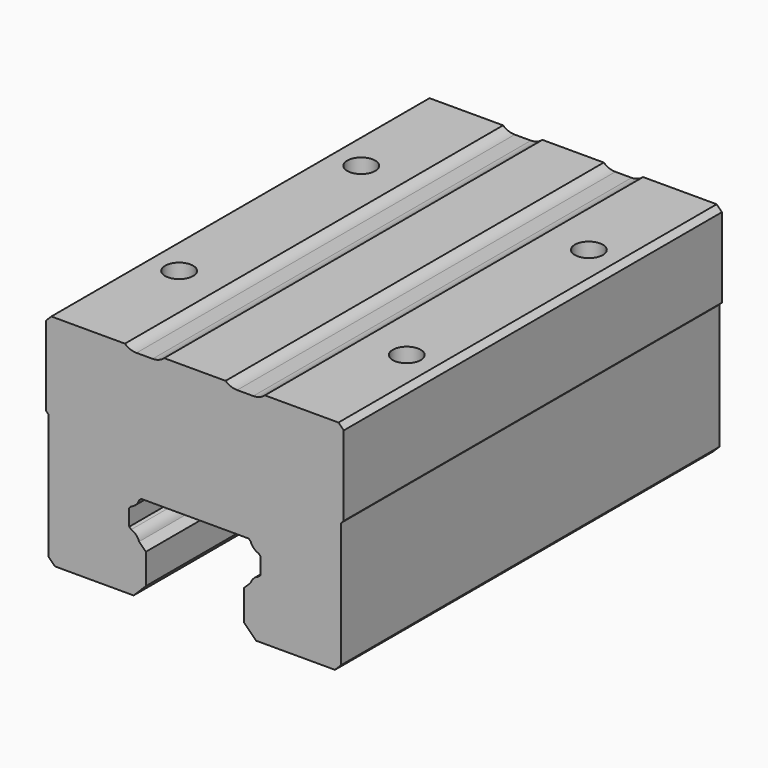
from build123d import *

# Parameters (mm, degrees)
F1_DEPTH = 54
F2_DEPTH = 54
F4_D     = 3.2
F4_DEPTH = 14.25
F4_TIP   = 0.9613769904


# Not quite as in the source:
# - ends of sketch curves that miss each other by under 0.0002 mm in the source are joined


with BuildPart() as f1:
    # F0 (on Front) → F1 (new body)
    with BuildSketch(Plane.XZ):
        with BuildLine():
            Line((-15.9999975914, -11.0858444687), (-13.9999981419, -11.0858444687))
            Line((-13.9999981419, -11.0858444687), (-14.9999975913, -10.0858455697))
            Line((-14.9999975913, -10.0858455697), (-14.9999975913, 8.4141544303))
            Line((-14.9999975913, 8.4141544303), (-13.9999975913, 9.4141544303))
            Line((-13.9999975913, 9.4141544303), (14.0000024087, 9.4141544303))
            Line((14.0000024087, 9.4141544303), (15.0000024087, 8.4141544303))
            Line((15.0000024087, 8.4141544303), (15.0000024087, -10.0858455697))
            Line((15.0000024087, -10.0858455697), (14.0000024087, -11.0858455697))
            Line((14.0000024087, -11.0858455697), (16.0000024087, -11.0858444685))
            Line((16.0000024087, -11.0858444685), (16.7000024086, -10.3858444685))
            Line((16.7000024086, -10.3858444685), (16.7000024087, 3.914155003))
            Line((16.7000024087, 3.914155003), (17.0000024087, 4.2141550029))
            Line((17.0000024087, 4.2141550029), (17.0000024088, 13.3141544304))
            Line((17.0000024088, 13.3141544304), (16.4000024089, 13.9141544303))
            Line((16.4000024089, 13.9141544303), (7.9944513482, 13.9141544304))
            ThreePointArc((7.9944513482, 13.9141544304), (7.3786811713, 13.5433235007), (6.671572232, 13.4141513784))
            Line((6.671572232, 13.4141513784), (4.8284325856, 13.4141513784))
            ThreePointArc((4.8284325856, 13.4141513784), (4.1213236463, 13.5433235007), (3.5055534694, 13.9141544304))
            Line((3.5055534694, 13.9141544304), (-3.5055486519, 13.9141544303))
            ThreePointArc((-3.5055486519, 13.9141544303), (-4.1213188288, 13.5433235006), (-4.828427768, 13.4141513784))
            Line((-4.828427768, 13.4141513784), (-6.6715674144, 13.4141513784))
            ThreePointArc((-6.6715674144, 13.4141513784), (-7.3788732943, 13.5428024468), (-7.9944465306, 13.9141544304))
            Line((-7.9944465306, 13.9141544304), (-16.3999975914, 13.9141544303))
            Line((-16.3999975914, 13.9141544303), (-16.9999975913, 13.3141544304))
            Line((-16.9999975913, 13.3141544304), (-16.9999975913, 4.2141550029))
            Line((-16.9999975913, 4.2141550029), (-16.6999975912, 3.9141550028))
            Line((-16.6999975912, 3.9141550028), (-16.6999975914, -10.3858444687))
            Line((-16.6999975914, -10.3858444687), (-15.9999975914, -11.0858444687))
        make_face()
    extrude(amount=-F1_DEPTH)

    # F0 (on Front) → F2 (join)
    with BuildSketch(Plane.XZ):
        with BuildLine():
            Line((-13.9999975913, -11.0858455697), (-6.9999968681, -11.0858455697))
            Line((-6.9999968681, -11.0858455697), (-5.5999972297, -9.6858459313))
            Line((-5.5999972297, -9.6858459313), (-5.5999972297, -6.2358522996))
            Line((-5.5999972297, -6.2358522996), (-6.3686160385, -5.4672334908))
            ThreePointArc((-6.3686160385, -5.4672334908), (-6.7178259107, -4.9036746123), (-7.2813847892, -4.5544647401))
            Line((-7.2813847892, -4.5544647401), (-7.4999972297, -4.3358522996))
            Line((-7.4999972297, -4.3358522996), (-7.4999972297, -2.435839563))
            Line((-7.4999972297, -2.435839563), (-7.2813847892, -2.2172271225))
            ThreePointArc((-7.2813847892, -2.2172271225), (-6.7178259107, -1.8680172504), (-6.3686160385, -1.3044583718))
            Line((-6.3686160385, -1.3044583718), (-6.150003598, -1.0858459313))
            Line((-6.150003598, -1.0858459313), (6.1500091386, -1.0858459313))
            Line((6.1500091386, -1.0858459313), (6.3686215791, -1.3044583718))
            ThreePointArc((6.3686215791, -1.3044583718), (6.7178314512, -1.8680172504), (7.2813903298, -2.2172271225))
            Line((7.2813903298, -2.2172271225), (7.5000027703, -2.435839563))
            Line((7.5000027703, -2.435839563), (7.5000027704, -4.3358522996))
            Line((7.5000027704, -4.3358522996), (7.2813903299, -4.5544647401))
            ThreePointArc((7.2813903299, -4.5544647401), (6.7178314513, -4.9036746123), (6.3686215792, -5.4672334908))
            Line((6.3686215792, -5.4672334908), (5.6000027704, -6.2358522996))
            Line((5.6000027704, -6.2358522996), (5.6000027703, -9.6858459313))
            Line((5.6000027703, -9.6858459313), (7.0000024087, -11.0858455697))
            Line((7.0000024087, -11.0858455697), (14.0000024087, -11.0858455697))
            Line((14.0000024087, -11.0858455697), (15.0000024087, -10.0858455697))
            Line((15.0000024087, -10.0858455697), (15.0000024087, 8.4141544303))
            Line((15.0000024087, 8.4141544303), (14.0000024087, 9.4141544303))
            Line((14.0000024087, 9.4141544303), (-13.9999975913, 9.4141544303))
            Line((-13.9999975913, 9.4141544303), (-14.9999975913, 8.4141544303))
            Line((-14.9999975913, 8.4141544303), (-14.9999975913, -10.0858455697))
            Line((-14.9999975913, -10.0858455697), (-13.9999975913, -11.0858455697))
        make_face()
    extrude(amount=-F2_DEPTH)

    # F4
    with Locations(Plane.XY.offset(13.9141544304)):
        with Locations((13.0000000001, 14), (-12.9999999999, 14), (-12.9999999999, 40), (13.0000000001, 40)):
            Hole(F4_D / 2, depth=F4_DEPTH)
            with Locations((0, 0, -(F4_DEPTH + F4_TIP / 2))):  # 118° drill point
                Cone(0, F4_D / 2, F4_TIP, mode=Mode.SUBTRACT)


solid = f1.part
